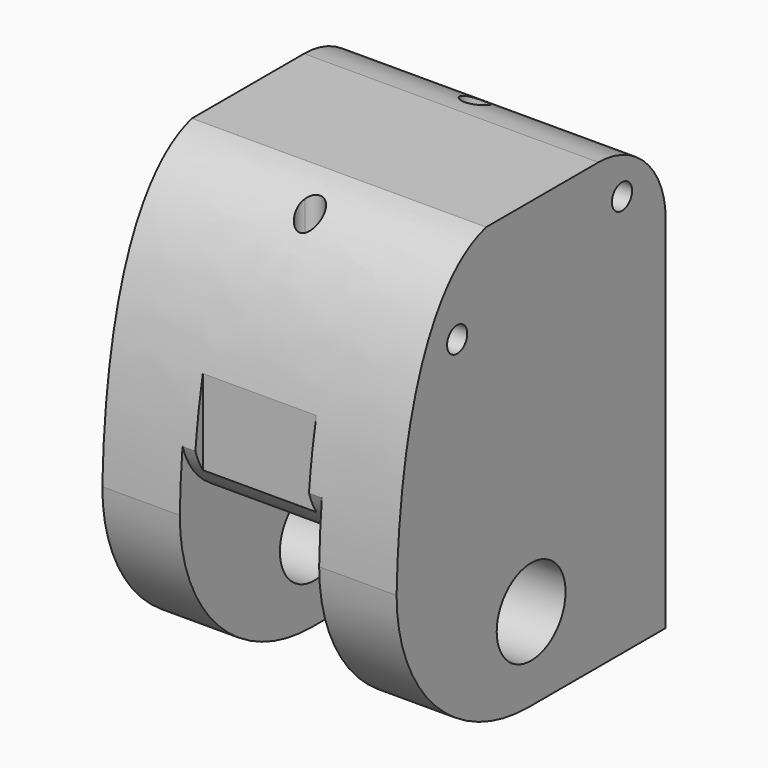
from build123d import *

# Parameters (mm, degrees)
F1_DEPTH  = 10.16
F2_R      = 2.6
F3_DEPTH  = 17.781
F4_R      = 10
F5_R      = 5
F7_DEPTH  = 17.781
F8_R      = 5.08
F10_DEPTH = 16.8384001672
F11_R     = 0.762
F12_DEPTH = 17.7810001
F16_DEPTH = 15.32
F17_DEPTH = 0.762


# Not quite as in the source:
# - an extrude ends at something that could not be found from the text; its depth is read off the source's solid
# - a feature names something its author has since deleted; it is built from what else it names


with BuildPart() as f1:
    # F0 (on Front) → F1 (new body, symmetric)
    with BuildSketch(Plane.XZ):
        Polygon((4.21, -13.4187000336), (8.89, -13.4187000336), (8.89, 13.4187000336), (-8.89, 13.4187000336), (-8.89, -13.4187000336), (-4.21, -13.4187000336), (-4.21, -3.4187000336), (4.21, -3.4187000336), align=None)
    extrude(amount=F1_DEPTH, both=True)

    # F2 (on face) → F3 (cut, through all)
    with BuildSketch(Plane(origin=(-8.89, 0, 0), x_dir=(0, -1, 0), z_dir=(-1, 0, 0))):
        with Locations((0, -8.4187000336)):
            Circle(F2_R)
    extrude(amount=-F3_DEPTH, mode=Mode.SUBTRACT)

    # F4
    f4_edges = [f1.edges().sort_by_distance(p)[0] for p in [
        (6.55, -10.16, -13.4187),
        (-6.55, -10.16, -13.4187),
    ]]
    fillet(f4_edges, radius=F4_R)

    # F5
    f5_edges = [f1.edges().sort_by_distance(p)[0] for p in [
        (0, -10.16, -3.4187),
    ]]
    fillet(f5_edges, radius=F5_R)

    # F6 (on face) → F7 (cut, through all)
    with BuildSketch(Plane(origin=(-8.89, 0, 0), x_dir=(0, -1, 0), z_dir=(-1, 0, 0))):
        with BuildLine():
            Line((10.16, -3.4187000336), (10.16, 13.4187000336))
            Line((10.16, 13.4187000336), (3.3866666667, 13.4187000336))
            add(Edge.make_bspline(
                [(3.3981708443, 13.4156480579), (3.3924205969, 13.4171809572), (3.3866666667, 13.4187000336)],
                knots=[0, 0, 0, 0.0008386489, 0.0008386489, 0.0008386489], degree=2, weights=[1, 0.9999999121, 1]))
            add(Edge.make_bspline(
                [(10.16, -3.4187000336), (9.7910592754, 11.7114337008), (3.3981708443, 13.4156480579)],
                knots=[5.4107177834, 5.4107177834, 5.4107177834, 6.2831853072, 6.2831853072, 6.2831853072], degree=2, weights=[1, 0.9063494321, 1]))
        make_face()
    extrude(amount=-F7_DEPTH, mode=Mode.SUBTRACT)

    # F8
    f8_edges = [f1.edges().sort_by_distance(p)[0] for p in [
        (0, 10.16, 13.4187),
    ]]
    fillet(f8_edges, radius=F8_R)

    # F9 (on face) → F10 (cut, through all)
    with BuildSketch(Plane(origin=(0, 0, -3.4187000336), x_dir=(1, 0, 0), z_dir=(0, 0, -1))):
        with BuildLine():
            Line((0.6304442878, 5.16), (-0.6304442878, 5.16))
            ThreePointArc((-0.6304442878, 5.16), (0, 4.826), (0.6304442878, 5.16))
        make_face()
        with BuildLine():
            ThreePointArc((0, 6.35), (-0.6733424092, 5.9447267862), (-0.6304442878, 5.16))
            Line((-0.6304442878, 5.16), (0.6304442878, 5.16))
            ThreePointArc((0.6304442878, 5.16), (0.7283689132, 5.364118946), (0.762, 5.588))
            ThreePointArc((0.762, 5.588), (0.5388153673, 6.1268153673), (0, 6.35))
        make_face()
        with BuildLine():
            ThreePointArc((0.762, -6.858), (-0.5388153673, -6.3191846327), (0, -7.62))
            ThreePointArc((0, -7.62), (0.5388153673, -7.3968153673), (0.762, -6.858))
        make_face()
    extrude(amount=-F10_DEPTH, mode=Mode.SUBTRACT)

    # F11 (on face) → F12 (cut, through all)
    with BuildSketch(Plane(origin=(-8.89, 0, 0), x_dir=(0, -1, 0), z_dir=(-1, 0, 0))):
        with BuildLine():
            ThreePointArc((-6.096, 10.8787000336), (-6.858, 11.6407000336), (-7.62, 10.8787000336))
            ThreePointArc((-7.62, 10.8787000336), (-6.858, 10.1167000336), (-6.096, 10.8787000336))
        make_face()
        with Locations((5.588, 8.3387000336)):
            Circle(F11_R)
    extrude(amount=-F12_DEPTH, mode=Mode.SUBTRACT)

    # F15 (on face) → F16 (cut, through all)
    with BuildSketch(Plane(origin=(0, 10.16, 0), x_dir=(-1, 0, 0), z_dir=(0, 1, 0))):
        with BuildLine():
            Line((0, -3.4187000336), (0, 1.6612999664))
            Line((0, 1.6612999664), (-3.448, 1.6612999664))
            ThreePointArc((-3.448, 1.6612999664), (-3.9868153673, 1.4381153337), (-4.21, 0.8992999664))
            Line((-4.21, 0.8992999664), (-4.21, -3.4187000336))
            Line((-4.21, -3.4187000336), (0, -3.4187000336))
        make_face()
        with BuildLine():
            Line((3.448, 1.6612999664), (0, 1.6612999664))
            Line((0, 1.6612999664), (0, -3.4187000336))
            Line((0, -3.4187000336), (4.21, -3.4187000336))
            Line((4.21, -3.4187000336), (4.21, 0.8992999664))
            ThreePointArc((4.21, 0.8992999664), (3.9868153673, 1.4381153337), (3.448, 1.6612999664))
        make_face()
    extrude(amount=-F16_DEPTH, mode=Mode.SUBTRACT)

    # F14 (on face) → F17 (cut)
    with BuildSketch(Plane.XZ.offset(10.16)):
        with BuildLine():
            Line((0, 6.9417000336), (3.429, 6.9417000336))
            ThreePointArc((3.429, 6.9417000336), (2.4246691527, 9.3663691863), (0, 10.3707000336))
            ThreePointArc((0, 10.3707000336), (-2.4246691527, 9.3663691863), (-3.429, 6.9417000336))
            Line((-3.429, 6.9417000336), (0, 6.9417000336))
        make_face()
        with BuildLine():
            ThreePointArc((-3.429, 6.9417000336), (0, 3.5127000336), (3.429, 6.9417000336))
            Line((3.429, 6.9417000336), (0, 6.9417000336))
            Line((0, 6.9417000336), (-3.429, 6.9417000336))
        make_face()
        with BuildLine():
            Line((3.429, -3.4187000336), (3.429, 6.9417000336))
            ThreePointArc((3.429, 6.9417000336), (0, 3.5127000336), (-3.429, 6.9417000336))
            Line((-3.429, 6.9417000336), (-3.429, -3.4187000336))
            Line((-3.429, -3.4187000336), (3.429, -3.4187000336))
        make_face()
    extrude(amount=-F17_DEPTH, mode=Mode.SUBTRACT)


solid = f1.part
